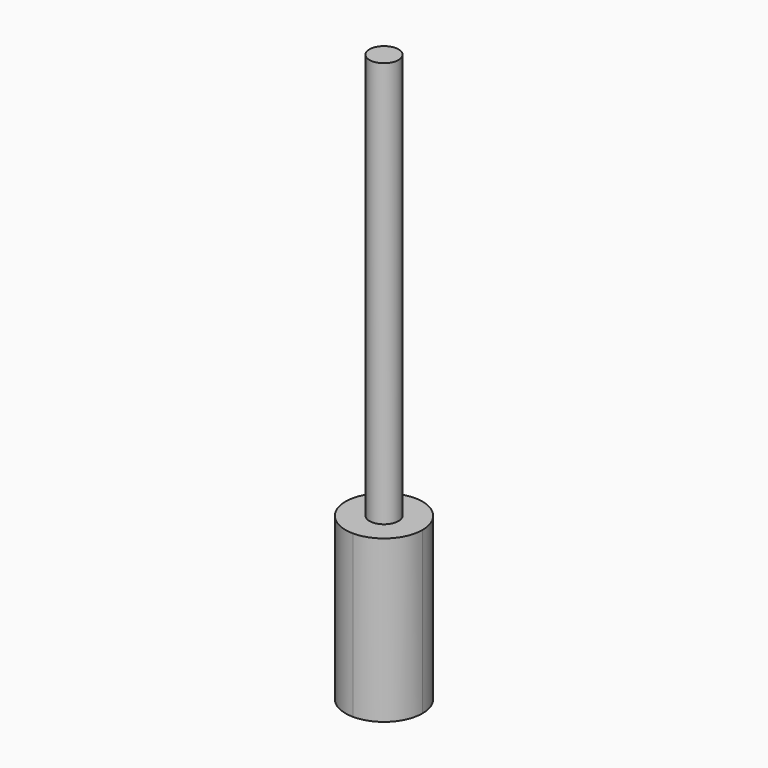
from build123d import *

# Parameters (mm, degrees)
F0_W        = 11.43
F0_H        = 11.43
F0_R        = 2.15265
F1_DEPTH    = 22.4125
F2_W        = 11.43
F2_H        = 11.43
F3_DEPTH    = 1.5875
F4_R        = 1.35255
F5_REACH    = 15.2565891076
F6_T1_DEPTH = 52.575
F7_R        = 2.15265
F8_DEPTH    = 60.325


# Not quite as in the source:
# - a fillet or chamfer that OpenCascade refuses, or shapes differently, is made with other operations: its cross-section is extruded or revolved along the edge and cut away or added


with BuildPart() as f1:
    # F0 (on Top) → F1 (new body)
    with BuildSketch(Plane.XY):
        Rectangle(F0_W, F0_H)
        Circle(F0_R, mode=Mode.SUBTRACT)
    extrude(amount=F1_DEPTH)

    # F2 (on face) → F3 (join)
    with BuildSketch(Plane.XY.offset(22.4125)):
        Rectangle(F2_W, F2_H)
    extrude(amount=F3_DEPTH)

    f5_end = f1.faces().sort_by_distance((-2.15265, 0, 11.20625))[0]
    # F4 (on face) → F5 (cut, up to a face of the model that its end follows)
    with BuildSketch(Plane(origin=(-5.715, 0, 0), x_dir=(0, -1, 0), z_dir=(-1, 0, 0))):
        with Locations((0, 11.20625)):
            Circle(F4_R)
    f5_long = extrude(amount=-F5_REACH, mode=Mode.PRIVATE)
    add(split(f5_long, bisect_by=f5_end, keep=Keep.ALL, mode=Mode.PRIVATE).solids().sort_by_distance((-5.715, 0, 11.20625))[0], mode=Mode.SUBTRACT)

    # F6: fillet of radius 5.715 on 4 edges, made by hand

    # F6_s2 → F6_t1 (cut)
    with BuildSketch(Plane.XY.offset(-14.2875)):
        with BuildLine():
            ThreePointArc((0, -5.715), (-4.0411152545, -4.0411152545), (-5.715, 0))
            Line((-5.715, 0), (-5.715, -5.715))
            Line((-5.715, -5.715), (0, -5.715))
        make_face()
        with BuildLine():
            ThreePointArc((0, -5.715), (4.0411152545, -4.0411152545), (5.715, 0))
            Line((5.715, 0), (5.715, -5.715))
            Line((5.715, -5.715), (0, -5.715))
        make_face()
        with BuildLine():
            ThreePointArc((-5.715, 0), (-4.0411152545, 4.0411152545), (0, 5.715))
            Line((0, 5.715), (-5.715, 5.715))
            Line((-5.715, 5.715), (-5.715, 0))
        make_face()
        with BuildLine():
            ThreePointArc((5.715, 0), (4.0411152545, 4.0411152545), (0, 5.715))
            Line((0, 5.715), (5.715, 5.715))
            Line((5.715, 5.715), (5.715, 0))
        make_face()
    extrude(amount=F6_T1_DEPTH, mode=Mode.SUBTRACT)

    # F7 (on face) → F8 (join)
    with BuildSketch(Plane.XY.offset(24)):
        Circle(F7_R)
    extrude(amount=F8_DEPTH)


solid = f1.part
